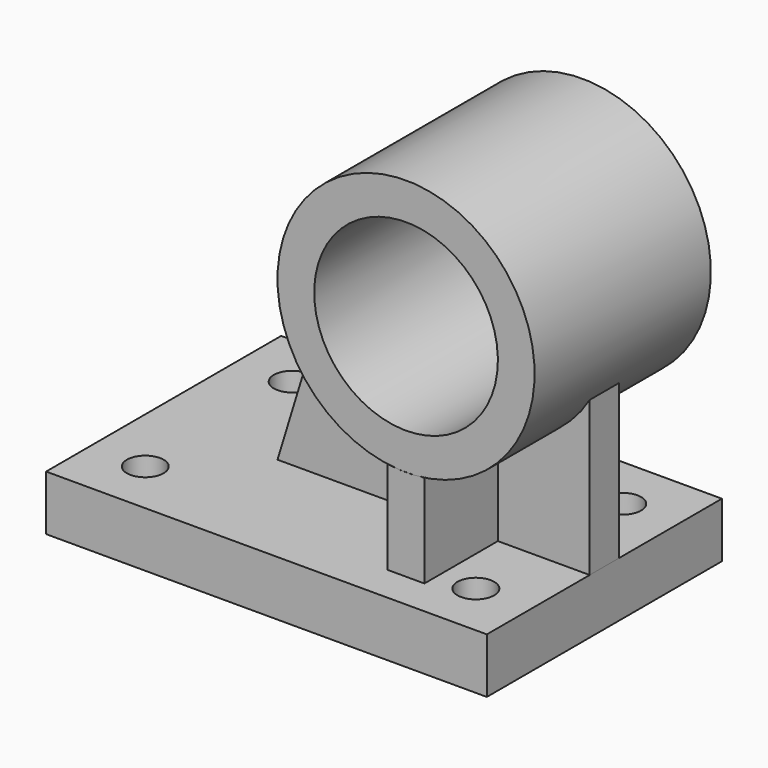
from build123d import *

# Parameters (mm, degrees)
F0_W          = 3048
F0_H          = 2032
F1_DEPTH      = 381
F2_R          = 127
F3_DEPTH      = 381.001
F6_DEPTH      = 762
F6_DEPTH_BACK = 762
F7_DEPTH      = 127
F7_DEPTH_BACK = 127
F8_DEPTH      = 762
F8_DEPTH_BACK = 762


# Not quite as in the source:
# - a feature names something its author has since deleted; it is built from what else it names


with BuildPart() as f1:
    # F0 (on Top) → F1 (new body)
    with BuildSketch(Plane.XY):
        with Locations((1524, 1016)):
            Rectangle(F0_W, F0_H)
    extrude(amount=F1_DEPTH)

    # F2 (on face) → F3 (cut, through all)
    with BuildSketch(Plane.XY.offset(381)):
        with Locations((381, 381)):
            Circle(F2_R)
        with Locations((2667, 1651)):
            Circle(F2_R)
        with Locations((2667, 381)):
            Circle(F2_R)
        with Locations((381, 1651)):
            Circle(F2_R)
    extrude(amount=-F3_DEPTH, mode=Mode.SUBTRACT)

    # F5 (on offset) → F8 (join, two sides)
    with BuildSketch(Plane.XZ.offset(-1016)) as f8_sk:
        with BuildLine():
            ThreePointArc((2413, 1025.118189755), (2286, 1016), (2159, 1025.118189755))
            Line((2159, 1025.118189755), (2159, 381))
            Line((2159, 381), (2413, 381))
            Line((2413, 381), (2413, 1025.118189755))
        make_face()
    extrude(amount=F8_DEPTH)
    extrude(f8_sk.sketch, amount=-F8_DEPTH_BACK)


with BuildPart() as f6:
    # F5 (on offset) → F6 (new body, two sides)
    with BuildSketch(Plane.XZ.offset(-1016)) as f6_sk:
        with BuildLine():
            ThreePointArc((3048, 1447.094988016), (3142.6618352652, 1667.4047559398), (3175, 1905))
            ThreePointArc((3175, 1905), (2417.7284143182, 2784.1863425129), (1436.0379643167, 2165.5485327097))
            Line((1436.0379643167, 2165.5485327097), (1690.1354455927, 2124.4776362207))
            ThreePointArc((1690.1354455927, 2124.4776362207), (2387.3228201241, 2531.8641687974), (2920.6663706387, 1925.5814960652))
            Line((2920.6663706387, 1925.5814960652), (3048, 1905))
            Line((3048, 1905), (3048, 1447.094988016))
        make_face()
        with BuildLine():
            Line((1690.1354455927, 2124.4776362207), (1436.0379643167, 2165.5485327097))
            ThreePointArc((1436.0379643167, 2165.5485327097), (1535.1611047805, 1429.0147550338), (2159, 1025.118189755))
            ThreePointArc((2159, 1025.118189755), (2286, 1016), (2413, 1025.118189755))
            ThreePointArc((2413, 1025.118189755), (2778.0328795595, 1164.5780625668), (3048, 1447.094988016))
            Line((3048, 1447.094988016), (3048, 1905))
            Line((3048, 1905), (2920.6663706387, 1925.5814960652))
            ThreePointArc((2920.6663706387, 1925.5814960652), (2920.9165871812, 1915.2920999902), (2921, 1905))
            ThreePointArc((2921, 1905), (2174.5302553349, 1279.8604187669), (1690.1354455927, 2124.4776362207))
        make_face()
    extrude(amount=F6_DEPTH)
    extrude(f6_sk.sketch, amount=-F6_DEPTH_BACK)


with BuildPart() as f7:
    # F5 (on offset) → F7 (new body, two sides)
    with BuildSketch(Plane.XZ.offset(-1016)) as f7_sk:
        with BuildLine():
            ThreePointArc((2413, 1025.118189755), (2286, 1016), (2159, 1025.118189755))
            Line((2159, 1025.118189755), (2159, 381))
            Line((2159, 381), (2413, 381))
            Line((2413, 381), (2413, 1025.118189755))
        make_face()
        with BuildLine():
            Line((3048, 381), (3048, 1447.094988016))
            ThreePointArc((3048, 1447.094988016), (2778.0328795595, 1164.5780625668), (2413, 1025.118189755))
            Line((2413, 1025.118189755), (2413, 381))
            Line((2413, 381), (3048, 381))
        make_face()
        with BuildLine():
            ThreePointArc((2159, 1025.118189755), (1535.1611047805, 1429.0147550338), (1436.0379643167, 2165.5485327097))
            Line((1436.0379643167, 2165.5485327097), (889, 381))
            Line((889, 381), (2159, 381))
            Line((2159, 381), (2159, 1025.118189755))
        make_face()
    extrude(amount=F7_DEPTH)
    extrude(f7_sk.sketch, amount=-F7_DEPTH_BACK)


solid = Compound([f1.part, f6.part, f7.part])
